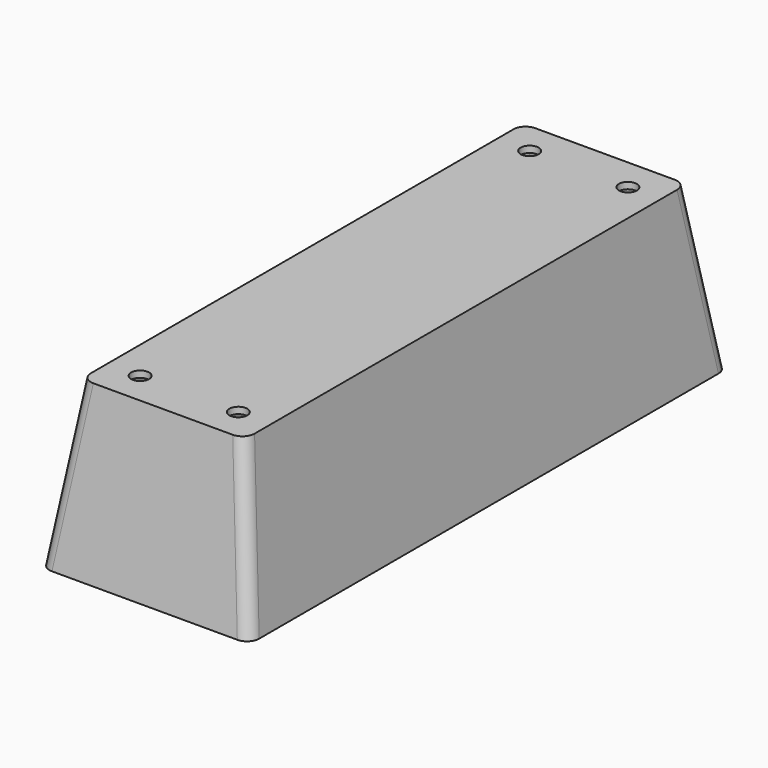
from build123d import *

# Parameters (mm, degrees)
F0_W                   = 40
F0_H                   = 135
F1_DEPTH               = 40
DRAFT_F1_DRAFTED_ANGLE = -8
F2_R                   = 3
F3_T                   = -1.584
F5_D                   = 4.4


# Not quite as in the source:
# - an extrude with a draft is written as a straight extrude whose walls are then drafted


with BuildPart() as f1:
    # F0 (on Top) → F1 (new body)
    with BuildSketch(Plane.XY):
        Rectangle(F0_W, F0_H)
    extrude(amount=-F1_DEPTH)

    # draft_F1_drafted
    draft_f1_drafted_walls = [f1.faces().sort_by_distance(p)[0] for p in [
        (20, 0, -26.6666666667),
        (0, 67.5, -26.6666666667),
        (-20, 0, -26.6666666667),
        (0, -67.5, -26.6666666667),
    ]]
    draft(draft_f1_drafted_walls, neutral_plane=Plane(origin=(0, 0, 0), x_dir=(1, 0, 0), z_dir=(0, 0, -1)), angle=DRAFT_F1_DRAFTED_ANGLE)

    # F2
    f2_edges = [f1.edges().sort_by_distance(p)[0] for p in [
        (22.810817, -70.310817, -20),
        (22.810817, 70.310817, -20),
        (-22.810817, 70.310817, -20),
        (-22.810817, -70.310817, -20),
    ]]
    fillet(f2_edges, radius=F2_R)

    # F3
    f3_openings = [f1.faces().sort_by_distance(p)[0] for p in [
        (0, 0, -40),
    ]]
    offset(amount=F3_T, openings=f3_openings, kind=Kind.INTERSECTION)

    # F5 (through all)
    with Locations(Plane.XY):
        with Locations((-12, 59.5), (-12, -59.5), (12, -59.5), (12, 59.5)):
            Hole(F5_D / 2)


solid = f1.part
